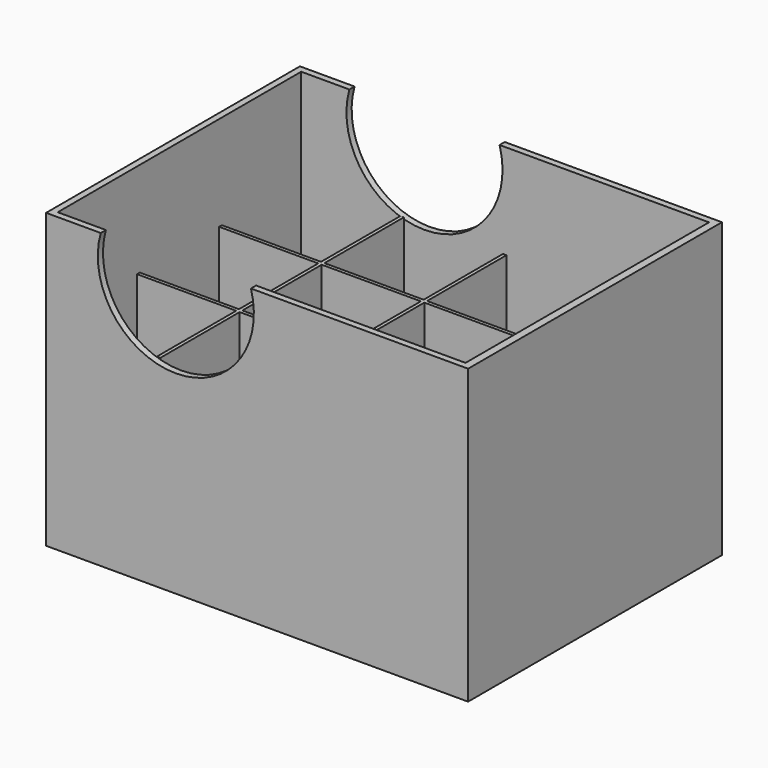
from build123d import *

# Parameters (mm, degrees)
F0_W     = 23
F0_H     = 23
F0_R     = 8.75
F1_DEPTH = 0.9
F0_W_2   = 97.9
F0_H_2   = 73.6
F2_DEPTH = 68
F3_DEPTH = 46
F5_DEPTH = 100


# Not quite as in the source:
# - a feature names something its author has since deleted; it is built from what else it names


with BuildPart() as f1:
    # F0 (on Top) → F1 (new body)
    with BuildSketch(Plane.XY):
        with Locations((-35.95, 23.8)):
            Rectangle(F0_W, F0_H)
        with Locations((-35.95, 23.8)):
            Circle(F0_R, mode=Mode.SUBTRACT)
    extrude(amount=F1_DEPTH)


with BuildPart() as f1b:
    # F0 (on Top) → F1, piece 2 (new body)
    with BuildSketch(Plane.XY):
        with Locations((-12.15, 23.8)):
            Rectangle(F0_W, F0_H)
        with Locations((-12.15, 23.8)):
            Circle(F0_R, mode=Mode.SUBTRACT)
    extrude(amount=F1_DEPTH)


with BuildPart() as f1c:
    # F0 (on Top) → F1, piece 3 (new body)
    with BuildSketch(Plane.XY):
        with Locations((11.65, 23.8)):
            Rectangle(F0_W, F0_H)
        with Locations((11.65, 23.8)):
            Circle(F0_R, mode=Mode.SUBTRACT)
    extrude(amount=F1_DEPTH)


with BuildPart() as f1d:
    # F0 (on Top) → F1, piece 4 (new body)
    with BuildSketch(Plane.XY):
        Polygon((46.95, 35.3), (23.95, 35.3), (23.95, -35.3), (47.15, -35.3), (47.15, 35.3), align=None)
    extrude(amount=F1_DEPTH)


with BuildPart() as f1e:
    # F0 (on Top) → F1, piece 5 (new body)
    with BuildSketch(Plane.XY):
        with Locations((11.65, 0)):
            Rectangle(F0_W, F0_H)
        with Locations((11.65, 0)):
            Circle(F0_R, mode=Mode.SUBTRACT)
    extrude(amount=F1_DEPTH)


with BuildPart() as f1f:
    # F0 (on Top) → F1, piece 6 (new body)
    with BuildSketch(Plane.XY):
        with Locations((-12.15, 0)):
            Rectangle(F0_W, F0_H)
        with Locations((-12.15, 0)):
            Circle(F0_R, mode=Mode.SUBTRACT)
    extrude(amount=F1_DEPTH)


with BuildPart() as f1g:
    # F0 (on Top) → F1, piece 7 (new body)
    with BuildSketch(Plane.XY):
        with Locations((-35.95, 0)):
            Rectangle(F0_W, F0_H)
        with Locations((-35.95, 0)):
            Circle(F0_R, mode=Mode.SUBTRACT)
    extrude(amount=F1_DEPTH)


with BuildPart() as f1h:
    # F0 (on Top) → F1, piece 8 (new body)
    with BuildSketch(Plane.XY):
        with Locations((-35.95, -23.8)):
            Rectangle(F0_W, F0_H)
        with Locations((-35.95, -23.8)):
            Circle(F0_R, mode=Mode.SUBTRACT)
    extrude(amount=F1_DEPTH)


with BuildPart() as f1i:
    # F0 (on Top) → F1, piece 9 (new body)
    with BuildSketch(Plane.XY):
        with Locations((-12.15, -23.8)):
            Rectangle(F0_W, F0_H)
        with Locations((-12.15, -23.8)):
            Circle(F0_R, mode=Mode.SUBTRACT)
    extrude(amount=F1_DEPTH)


with BuildPart() as f1j:
    # F0 (on Top) → F1, piece 10 (new body)
    with BuildSketch(Plane.XY):
        with Locations((11.65, -23.8)):
            Rectangle(F0_W, F0_H)
        with Locations((11.65, -23.8)):
            Circle(F0_R, mode=Mode.SUBTRACT)
    extrude(amount=F1_DEPTH)


with BuildPart() as f2:
    # F0 (on Top) → F2 (new body)
    with BuildSketch(Plane.XY):
        Rectangle(F0_W_2, F0_H_2)
        Polygon((23.15, 35.3), (23.95, 35.3), (46.95, 35.3), (47.15, 35.3), (47.15, -35.3), (23.95, -35.3), (23.15, -35.3), (0.15, -35.3), (-0.65, -35.3), (-23.65, -35.3), (-24.45, -35.3), (-47.45, -35.3), (-47.45, -12.3), (-47.45, -11.5), (-47.45, 11.5), (-47.45, 12.3), (-47.45, 35.3), (-24.45, 35.3), (-23.65, 35.3), (-0.65, 35.3), (0.15, 35.3), align=None, mode=Mode.SUBTRACT)
    extrude(amount=F2_DEPTH)

    # F4 (on face) → F5 (cut)
    with BuildSketch(Plane.XZ.offset(36.8)):
        with BuildLine():
            Line((-1.4258787883, 68), (-36.2741212117, 68))
            ThreePointArc((-36.2741212117, 68), (-18.85, 45), (-1.4258787883, 68))
        make_face()
    extrude(amount=-F5_DEPTH, mode=Mode.SUBTRACT)


with BuildPart() as f3:
    # F0 (on Top) → F3 (new body)
    with BuildSketch(Plane.XY):
        Polygon((23.95, -35.3), (23.95, 35.3), (23.15, 35.3), (23.15, 12.3), (0.15, 12.3), (0.15, 35.3), (-0.65, 35.3), (-0.65, 12.3), (-23.65, 12.3), (-23.65, 35.3), (-24.45, 35.3), (-24.45, 12.3), (-47.45, 12.3), (-47.45, 11.5), (-24.45, 11.5), (-24.45, -11.5), (-47.45, -11.5), (-47.45, -12.3), (-24.45, -12.3), (-24.45, -35.3), (-23.65, -35.3), (-23.65, -12.3), (-0.65, -12.3), (-0.65, -35.3), (0.15, -35.3), (0.15, -12.3), (23.15, -12.3), (23.15, -35.3), align=None)
        with Locations((-12.15, 0)):
            Rectangle(F0_W, F0_H, mode=Mode.SUBTRACT)
        with Locations((11.65, 0)):
            Rectangle(F0_W, F0_H, mode=Mode.SUBTRACT)
    extrude(amount=F3_DEPTH)


solid = Compound([f1.part, f1b.part, f1c.part, f1d.part, f1e.part, f1f.part, f1g.part, f1h.part, f1i.part, f1j.part, f2.part, f3.part])
